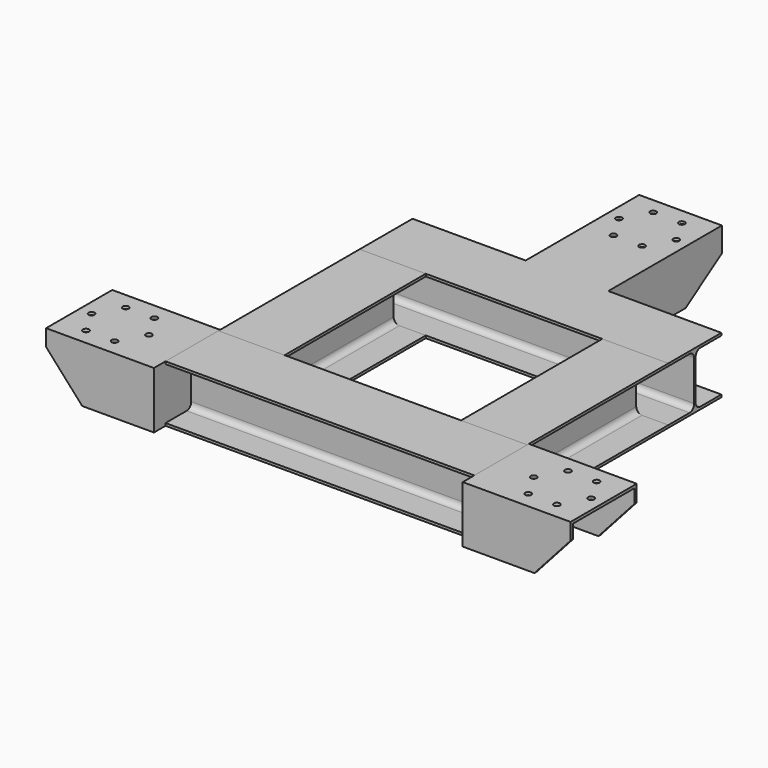
from build123d import *

# Parameters (mm, degrees)
F3_DEPTH  = 1120
F5_DEPTH  = 640
F8_DEPTH  = 9
F10_DEPTH = 10
F12_DEPTH = 10
F14_DEPTH = 10
F15_W     = 300
F15_H     = 10
F16_DEPTH = 381.073
F18_DEPTH = 10
F20_DEPTH = 10
F22_R     = 11
F23_DEPTH = 25


with BuildPart() as f3:
    # F2 (on line) → F3 (new body)
    with BuildSketch(Plane(origin=(560, 0, 0), x_dir=(0, -1, 0), z_dir=(-1, 0, 0))):
        with BuildLine():
            Line((560, -9), (560, 0))
            Line((560, 0), (320, 0))
            Line((320, 0), (320, -9))
            Line((320, -9), (415.75, -9))
            ThreePointArc((415.75, -9), (430.5992424049, -15.1507575951), (436.75, -30))
            Line((436.75, -30), (436.75, -176))
            ThreePointArc((436.75, -176), (430.5992424049, -190.8492424049), (415.75, -197))
            Line((415.75, -197), (320, -197))
            Line((320, -197), (320, -206))
            Line((320, -206), (560, -206))
            Line((560, -206), (560, -197))
            Line((560, -197), (464.25, -197))
            ThreePointArc((464.25, -197), (449.4007575951, -190.8492424049), (443.25, -176))
            Line((443.25, -176), (443.25, -30))
            ThreePointArc((443.25, -30), (449.4007575951, -15.1507575951), (464.25, -9))
            Line((464.25, -9), (560, -9))
        make_face()
    extrude(amount=F3_DEPTH)


with BuildPart() as f3b:
    # F2 (on line) → F3, piece 2 (new body)
    with BuildSketch(Plane(origin=(560, 0, 0), x_dir=(0, -1, 0), z_dir=(-1, 0, 0))):
        with BuildLine():
            Line((-320, 0), (-560, 0))
            Line((-560, 0), (-560, -9))
            Line((-560, -9), (-464.25, -9))
            ThreePointArc((-464.25, -9), (-449.4007575951, -15.1507575951), (-443.25, -30))
            Line((-443.25, -30), (-443.25, -176))
            ThreePointArc((-443.25, -176), (-449.4007575951, -190.8492424049), (-464.25, -197))
            Line((-464.25, -197), (-560, -197))
            Line((-560, -197), (-560, -206))
            Line((-560, -206), (-320, -206))
            Line((-320, -206), (-320, -197))
            Line((-320, -197), (-415.75, -197))
            ThreePointArc((-415.75, -197), (-430.5992424049, -190.8492424049), (-436.75, -176))
            Line((-436.75, -176), (-436.75, -30))
            ThreePointArc((-436.75, -30), (-430.5992424049, -15.1507575951), (-415.75, -9))
            Line((-415.75, -9), (-320, -9))
            Line((-320, -9), (-320, 0))
        make_face()
    extrude(amount=F3_DEPTH)

    # F7 (on face) → F8 (join)
    with BuildSketch(Plane.XY):
        Polygon((-150, 925.0000017314), (-150, 560), (150, 560), (150, 925.0000017314), (150, 1075.0000017314), (-150, 1075.0000017314), align=None)
    extrude(amount=-F8_DEPTH)

    # F9 (on face) → F10 (join)
    with BuildSketch(Plane(origin=(-150, 0, 0), x_dir=(0, -1, 0), z_dir=(-1, 0, 0))):
        with BuildLine():
            Line((-464.25, -9), (-560, -9))
            Line((-560, -9), (-1075.0000017314, -9))
            Line((-1075.0000017314, -9), (-1075.0000017314, -89))
            Line((-1075.0000017314, -89), (-910, -197))
            Line((-910, -197), (-560, -197))
            Line((-560, -197), (-464.25, -197))
            ThreePointArc((-464.25, -197), (-449.4007575951, -190.8492424049), (-443.25, -176))
            Line((-443.25, -176), (-443.25, -30))
            ThreePointArc((-443.25, -30), (-449.4007575951, -15.1507575951), (-464.25, -9))
        make_face()
    extrude(amount=-F10_DEPTH)

    # F11 (on face) → F12 (join)
    with BuildSketch(Plane.YZ.offset(150)):
        with BuildLine():
            Line((1075.0000017314, -9), (560, -9))
            Line((560, -9), (464.25, -9))
            ThreePointArc((464.25, -9), (449.4007575951, -15.1507575951), (443.25, -30))
            Line((443.25, -30), (443.25, -176))
            ThreePointArc((443.25, -176), (449.4007575951, -190.8492424049), (464.25, -197))
            Line((464.25, -197), (560, -197))
            Line((560, -197), (910, -197))
            Line((910, -197), (1075.0000017314, -89))
            Line((1075.0000017314, -89), (1075.0000017314, -9))
        make_face()
    extrude(amount=-F12_DEPTH)


with BuildPart() as f5:
    # F4 (on face) → F5 (new body, through all)
    with BuildSketch(Plane.XZ.offset(-320)):
        with BuildLine():
            Line((-320, 0), (-560, 0))
            Line((-560, 0), (-560, -9))
            Line((-560, -9), (-464.25, -9))
            ThreePointArc((-464.25, -9), (-449.4007575951, -15.1507575951), (-443.25, -30))
            Line((-443.25, -30), (-443.25, -176))
            ThreePointArc((-443.25, -176), (-449.4007575951, -190.8492424049), (-464.25, -197))
            Line((-464.25, -197), (-560, -197))
            Line((-560, -197), (-560, -206))
            Line((-560, -206), (-320, -206))
            Line((-320, -206), (-320, -197))
            Line((-320, -197), (-415.75, -197))
            ThreePointArc((-415.75, -197), (-430.5992424049, -190.8492424049), (-436.75, -176))
            Line((-436.75, -176), (-436.75, -30))
            ThreePointArc((-436.75, -30), (-430.5992424049, -15.1507575951), (-415.75, -9))
            Line((-415.75, -9), (-320, -9))
            Line((-320, -9), (-320, 0))
        make_face()
    extrude(amount=F5_DEPTH)


with BuildPart() as f5b:
    # F4 (on face) → F5, piece 2 (new body, through all)
    with BuildSketch(Plane.XZ.offset(-320)):
        with BuildLine():
            Line((560, -206), (560, -197))
            Line((560, -197), (464.25, -197))
            ThreePointArc((464.25, -197), (449.4007575951, -190.8492424049), (443.25, -176))
            Line((443.25, -176), (443.25, -30))
            ThreePointArc((443.25, -30), (449.4007575951, -15.1507575951), (464.25, -9))
            Line((464.25, -9), (560, -9))
            Line((560, -9), (560, 0))
            Line((560, 0), (320, 0))
            Line((320, 0), (320, -9))
            Line((320, -9), (415.75, -9))
            ThreePointArc((415.75, -9), (430.5992424049, -15.1507575951), (436.75, -30))
            Line((436.75, -30), (436.75, -176))
            ThreePointArc((436.75, -176), (430.5992424049, -190.8492424049), (415.75, -197))
            Line((415.75, -197), (320, -197))
            Line((320, -197), (320, -206))
            Line((320, -206), (560, -206))
        make_face()
    extrude(amount=F5_DEPTH)


with BuildPart() as f14:
    # F13 (on face) → F14 (new body)
    with BuildSketch(Plane(origin=(-560, 0, 0), x_dir=(0, -1, 0), z_dir=(-1, 0, 0))):
        with BuildLine():
            Line((312.5000008657, 0), (312.5000008657, -206))
            Line((312.5000008657, -206), (320, -206))
            Line((320, -206), (320, -197))
            Line((320, -197), (415.75, -197))
            ThreePointArc((415.75, -197), (430.5992424049, -190.8492424049), (436.75, -176))
            Line((436.75, -176), (436.75, -30))
            ThreePointArc((436.75, -30), (430.5992424049, -15.1507575951), (415.75, -9))
            Line((415.75, -9), (320, -9))
            Line((320, -9), (320, 0))
            Line((320, 0), (312.5000008657, 0))
        make_face()
        with BuildLine():
            Line((320, -197), (320, -206))
            Line((320, -206), (560, -206))
            Line((560, -206), (560, -197))
            Line((560, -197), (464.25, -197))
            ThreePointArc((464.25, -197), (449.4007575951, -190.8492424049), (443.25, -176))
            Line((443.25, -176), (443.25, -30))
            ThreePointArc((443.25, -30), (449.4007575951, -15.1507575951), (464.25, -9))
            Line((464.25, -9), (560, -9))
            Line((560, -9), (560, 0))
            Line((560, 0), (462.5000008657, 0))
            Line((462.5000008657, 0), (320, 0))
            Line((320, 0), (320, -9))
            Line((320, -9), (415.75, -9))
            ThreePointArc((415.75, -9), (430.5992424049, -15.1507575951), (436.75, -30))
            Line((436.75, -30), (436.75, -176))
            ThreePointArc((436.75, -176), (430.5992424049, -190.8492424049), (415.75, -197))
            Line((415.75, -197), (320, -197))
        make_face()
        with BuildLine():
            Line((560, -197), (560, -206))
            Line((560, -206), (612.5000008657, -206))
            Line((612.5000008657, -206), (612.5000008657, 0))
            Line((612.5000008657, 0), (560, 0))
            Line((560, 0), (560, -9))
            Line((560, -9), (464.25, -9))
            ThreePointArc((464.25, -9), (449.4007575951, -15.1507575951), (443.25, -30))
            Line((443.25, -30), (443.25, -176))
            ThreePointArc((443.25, -176), (449.4007575951, -190.8492424049), (464.25, -197))
            Line((464.25, -197), (560, -197))
        make_face()
    extrude(amount=F14_DEPTH)

    # F15 (on face) → F16 (join)
    with BuildSketch(Plane(origin=(-570, 0, 0), x_dir=(0, -1, 0), z_dir=(-1, 0, 0))):
        with Locations((462.5000008657, -5)):
            Rectangle(F15_W, F15_H)
    extrude(amount=F16_DEPTH)

    # F17 (on face) → F18 (join)
    with BuildSketch(Plane(origin=(0, -312.5000008657, 0), x_dir=(-1, 0, 0), z_dir=(0, 1, 0))):
        Polygon((951.073, -60), (951.073, -10), (570, -10), (570, -206), (820, -206), align=None)
    extrude(amount=-F18_DEPTH)

    # F19 (on face) → F20 (join)
    with BuildSketch(Plane.XZ.offset(612.5000008657)):
        Polygon((-820, -206), (-570, -206), (-570, -10), (-951.073, -10), (-951.073, -60), align=None)
    extrude(amount=-F20_DEPTH)


with BuildPart() as f21_1:
    # F21: instance of F14
    add(f14.part.mirror(Plane.YZ))


with BuildPart() as f23_tool:
    # F22 (on face) → F23 (new body)
    with BuildSketch(Plane.XY):
        with Locations((104, 925.9345531464)):
            Circle(F22_R)
        with Locations((-853.8828452665, -372.9006345796)):
            Circle(F22_R)
        with Locations((749.8828452665, -553.0339185668)):
            Circle(F22_R)
        with Locations((-104, 925.9345531464)):
            Circle(F22_R)
        with Locations((-52, 1016.0011951399)):
            Circle(F22_R)
        with Locations((-52, 835.8679111528)):
            Circle(F22_R)
        with Locations((52, 1016.0011951399)):
            Circle(F22_R)
        with Locations((52, 835.8679111528)):
            Circle(F22_R)
        with Locations((-905.8828452665, -462.9672765732)):
            Circle(F22_R)
        with Locations((-697.8828452665, -462.9672765732)):
            Circle(F22_R)
        with Locations((-853.8828452665, -553.0339185668)):
            Circle(F22_R)
        with Locations((-749.8828452665, -553.0339185668)):
            Circle(F22_R)
        with Locations((-749.8828452665, -372.9006345796)):
            Circle(F22_R)
        with Locations((853.8828452665, -553.0339185668)):
            Circle(F22_R)
        with Locations((749.8828452665, -372.9006345796)):
            Circle(F22_R)
        with Locations((905.8828452665, -462.9672765732)):
            Circle(F22_R)
        with Locations((853.8828452665, -372.9006345796)):
            Circle(F22_R)
        with Locations((697.8828452665, -462.9672765732)):
            Circle(F22_R)
    extrude(amount=-F23_DEPTH)


with BuildPart() as f3b_1:
    add(f3b.part)

    # F23: cut by f23_tool
    add(f23_tool.part, mode=Mode.SUBTRACT)


with BuildPart() as f14_1:
    add(f14.part)

    # F23: cut by f23_tool
    add(f23_tool.part, mode=Mode.SUBTRACT)


with BuildPart() as f21_1_1:
    add(f21_1.part)

    # F23: cut by f23_tool
    add(f23_tool.part, mode=Mode.SUBTRACT)


solid = Compound([f3.part, f5.part, f5b.part, f3b_1.part, f14_1.part, f21_1_1.part])
